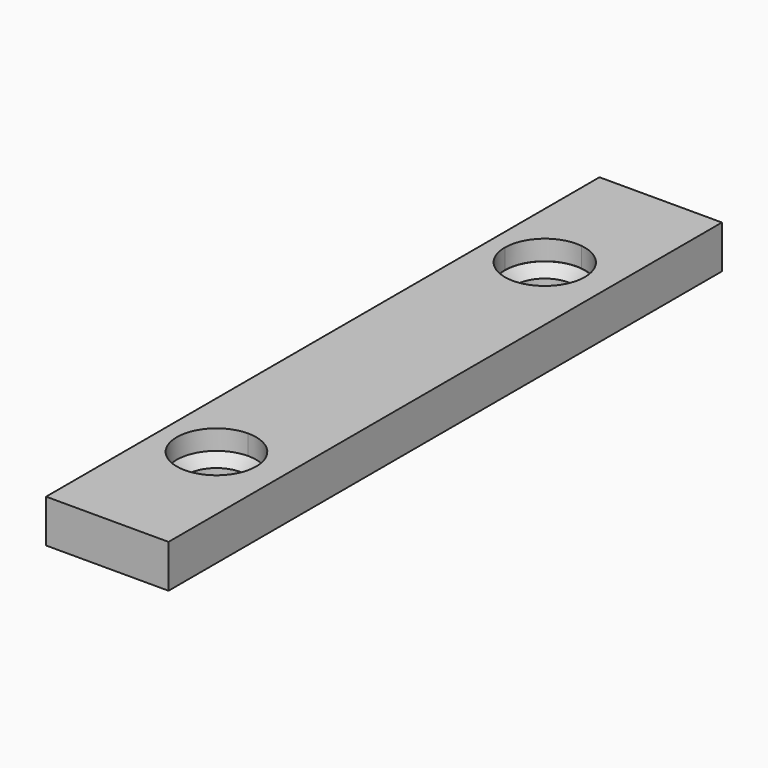
from build123d import *

# Parameters (mm, degrees)
F0_W           = 18.5
F0_H           = 104.5
F1_DEPTH       = 6.5
F3_DEPTH       = 3
F5_D           = 9
F5_CSINK_D     = 12
F5_CSINK_ANGLE = 90
F7_D           = 9
F7_CSINK_D     = 12
F7_CSINK_ANGLE = 90


with BuildPart() as f1:
    # F0 (on Top) → F1 (new body)
    with BuildSketch(Plane.XY):
        Rectangle(F0_W, F0_H)
    extrude(amount=F1_DEPTH)

    # F2 (on face) → F3 (cut)
    with BuildSketch(Plane.XY.offset(6.5)):
        with BuildLine():
            ThreePointArc((5.3333333333, 31.25), (3.8072646337, 35.2638648596), (0, 37.25))
            Line((0, 37.25), (0, 31.25))
            Line((0, 31.25), (5.3333333333, 31.25))
        make_face()
        with BuildLine():
            Line((0, 31.25), (0, 37.25))
            ThreePointArc((0, 37.25), (-4.7221981929, 35.765597967), (-6.75, 31.25))
            Line((-6.75, 31.25), (-0.7083333333, 31.25))
            Line((-0.7083333333, 31.25), (0, 31.25))
        make_face()
        with BuildLine():
            Line((5.3333333333, 31.25), (0, 31.25))
            Line((0, 31.25), (0, 25.25))
            ThreePointArc((0, 25.25), (3.8072646337, 27.2361351404), (5.3333333333, 31.25))
        make_face()
        with BuildLine():
            Line((0, 25.25), (0, 31.25))
            Line((0, 31.25), (-0.7083333333, 31.25))
            Line((-0.7083333333, 31.25), (-0.7083333333, 25.2083333333))
            ThreePointArc((-0.7083333333, 25.2083333333), (-0.3535544507, 25.2187589954), (0, 25.25))
        make_face()
        with BuildLine():
            Line((-0.7083333333, 31.25), (-6.75, 31.25))
            ThreePointArc((-6.75, 31.25), (-4.980436803, 26.9778965303), (-0.7083333333, 25.2083333333))
            Line((-0.7083333333, 25.2083333333), (-0.7083333333, 31.25))
        make_face()
        with BuildLine():
            ThreePointArc((5.2916666667, -30.75), (3.5343073538, -26.5073593129), (-0.7083333333, -24.75))
            Line((-0.7083333333, -24.75), (-0.7083333333, -36.75))
            ThreePointArc((-0.7083333333, -36.75), (3.5343073538, -34.9926406871), (5.2916666667, -30.75))
        make_face()
        with BuildLine():
            Line((-0.7083333333, -36.75), (-0.7083333333, -24.75))
            ThreePointArc((-0.7083333333, -24.75), (-6.7083333333, -30.75), (-0.7083333333, -36.75))
        make_face()
    extrude(amount=-F3_DEPTH, mode=Mode.SUBTRACT)

    # F5 (through all)
    with Locations(Plane.XY.offset(3.5)):
        with Locations((-0.7083333333, 31.25)):
            CounterSinkHole(F5_D / 2, F5_CSINK_D / 2, counter_sink_angle=F5_CSINK_ANGLE)

    # F7 (through all)
    with Locations(Plane.XY.offset(3.5)):
        with Locations((-0.7083333333, -30.75)):
            CounterSinkHole(F7_D / 2, F7_CSINK_D / 2, counter_sink_angle=F7_CSINK_ANGLE)


solid = f1.part
